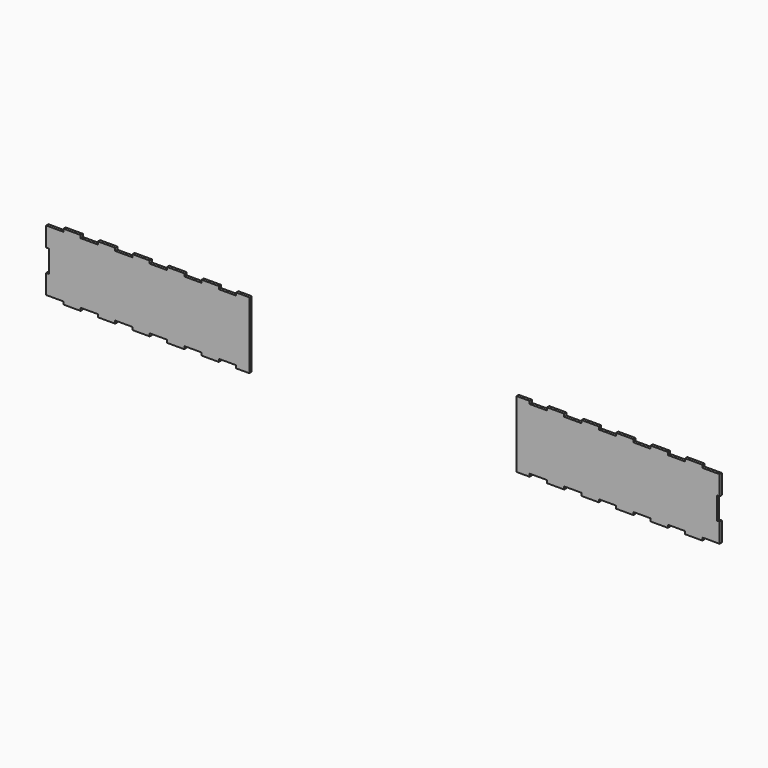
from build123d import *

# Parameters (mm, degrees)
F1_DEPTH = 3.175


# Not quite as in the source:
# - ends of sketch curves that miss each other by under 0.0002 mm in the source are joined


with BuildPart() as f1:
    # F0 (on Front) → F1 (new body)
    with BuildSketch(Plane.XZ):
        Polygon((-384.175, 34.925), (-384.175, 12.7), (-381, 12.7), (-381, -12.7), (-384.175, -12.7), (-384.175, -34.925), (-364.473717838, -34.925), (-364.473717838, -38.1), (-344.772435676, -38.1), (-344.772435676, -34.925), (-325.071153514, -34.925), (-325.071153514, -38.1), (-305.369871352, -38.1), (-305.369871352, -34.925), (-285.66858919, -34.925), (-285.66858919, -38.1), (-265.967307028, -38.1), (-265.967307028, -34.925), (-246.266024866, -34.925), (-246.266024866, -38.1), (-226.564742704, -38.1), (-226.564742704, -34.925), (-206.863460542, -34.925), (-206.863460542, -38.1), (-187.16217838, -38.1), (-187.16217838, -34.925), (-167.460896218, -34.925), (-167.460896218, -38.1), (-152.4, -38.1), (-152.4, 38.1), (-167.460896218, 38.1), (-167.460896218, 34.925), (-187.16217838, 34.925), (-187.16217838, 38.1), (-206.863460542, 38.1), (-206.863460542, 34.925), (-226.564742704, 34.925), (-226.564742704, 38.1), (-246.266024866, 38.1), (-246.266024866, 34.925), (-265.967307028, 34.925), (-265.967307028, 38.1), (-285.66858919, 38.1), (-285.66858919, 34.925), (-305.369871352, 34.925), (-305.369871352, 38.1), (-325.071153514, 38.1), (-325.071153514, 34.925), (-344.772435676, 34.925), (-344.772435676, 38.1), (-364.473717838, 38.1), (-364.473717838, 34.925), align=None)
    extrude(amount=F1_DEPTH)


with BuildPart() as f1b:
    # F0 (on Front) → F1, piece 2 (new body)
    with BuildSketch(Plane.XZ):
        Polygon((167.460900536, 38.1), (152.4, 38.1), (152.4, -38.1), (167.460900536, -38.1), (167.460900536, -34.925), (187.162182698, -34.925), (187.162182698, -38.1), (206.86346486, -38.1), (206.86346486, -34.925), (226.564747022, -34.925), (226.564747022, -38.1), (246.266029184, -38.1), (246.266029184, -34.925), (265.967311346, -34.925), (265.967311346, -38.1), (285.668593508, -38.1), (285.668593508, -34.925), (305.36987567, -34.925), (305.36987567, -38.1), (325.071157832, -38.1), (325.071157832, -34.925), (344.772439994, -34.925), (344.772439994, -38.1), (364.473722156, -38.1), (364.473722156, -34.925), (384.175004318, -34.925), (384.175, -12.7), (381, -12.7), (381, 12.7), (384.175, 12.7), (384.175, 34.925), (364.473722156, 34.925), (364.473722156, 38.1), (344.772439994, 38.1), (344.772439994, 34.925), (325.071157832, 34.925), (325.071157832, 38.1), (305.36987567, 38.1), (305.36987567, 34.925), (285.668593508, 34.925), (285.668593508, 38.1), (265.967311346, 38.1), (265.967311346, 34.925), (246.266029184, 34.925), (246.266029184, 38.1), (226.564747022, 38.1), (226.564747022, 34.925), (206.86346486, 34.925), (206.86346486, 38.1), (187.162182698, 38.1), (187.162182698, 34.925), (167.460900536, 34.925), align=None)
    extrude(amount=F1_DEPTH)


solid = Compound([f1.part, f1b.part])
